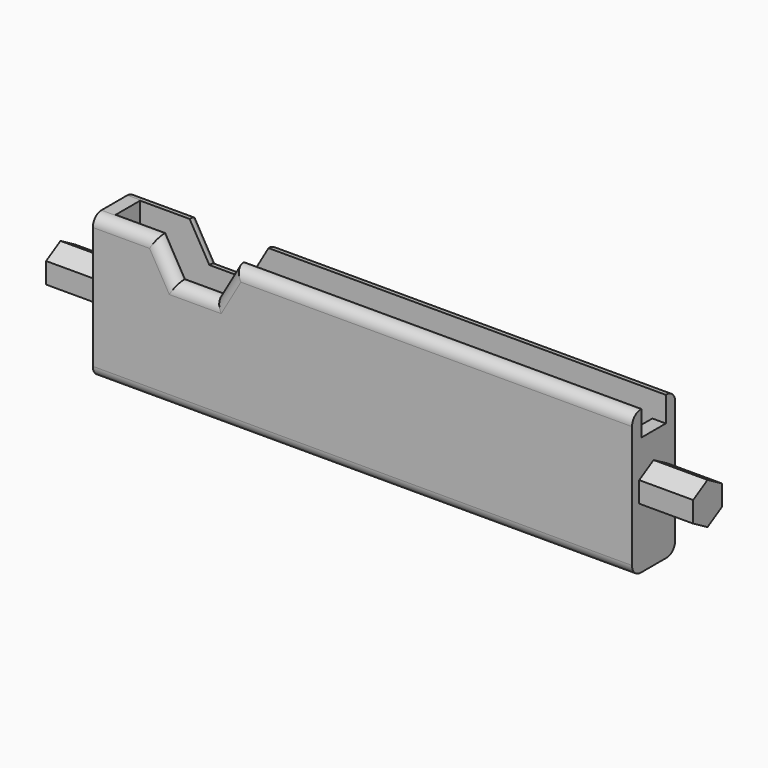
from build123d import *

# Parameters (mm, degrees)
F1_DEPTH = 7.5
F2_W     = 10
F2_H     = 42
F3_DEPTH = 4.25
F6_DEPTH = 15
F8_R     = 3


with BuildPart() as f1:
    # F0 (on Front) → F1 (new body, symmetric)
    with BuildSketch(Plane.XZ):
        Polygon((75, -20), (75, 20), (-35.5303448854, 20), (-41.0151724427, 10.5), (-51.9848275573, 10.5), (-57.4696551146, 20), (-75, 20), (-75, -20), align=None)
    extrude(amount=F1_DEPTH, both=True)

    # F2 (on Front) → F3 (cut, symmetric)
    with BuildSketch(Plane.XZ):
        Polygon((71.25, 13), (71.25, 55), (-71.25, 55), (-71.25, -15), (71.25, -15), align=None)
        with Locations((76.25, 34)):
            Rectangle(F2_W, F2_H)
    extrude(amount=F3_DEPTH, both=True, mode=Mode.SUBTRACT)



with BuildPart() as f6:
    # F5 (on offset) → F6 (new body)
    with BuildSketch(Plane.YZ.offset(75)):
        Polygon((5, -2.8867513459), (5, 2.8867513459), (0, 5.7735026919), (-5, 2.8867513459), (-5, -2.8867513459), (0, -5.7735026919), align=None)
    extrude(amount=F6_DEPTH)


with BuildPart() as f1_1:
    add(f1.part)

    add(f6.part)  # F7 merges F6
    # F7: F6 across plane
    add(f6.part.mirror(Plane.YZ))

    # F8
    f8_edges = [f1_1.edges().sort_by_distance(p)[0] for p in [
        (0, -7.5, -20),
        (0, 7.5, -20),
        (19.734828, -7.5, 20),
        (-66.234828, -7.5, 20),
        (-66.234828, 7.5, 20),
        (19.734828, 7.5, 20),
        (-54.727241, -7.5, 15.25),
        (-46.5, -7.5, 10.5),
        (-38.272759, -7.5, 15.25),
        (-38.272759, 7.5, 15.25),
        (-46.5, 7.5, 10.5),
        (-54.727241, 7.5, 15.25),
    ]]
    fillet(f8_edges, radius=F8_R)


solid = f1_1.part
